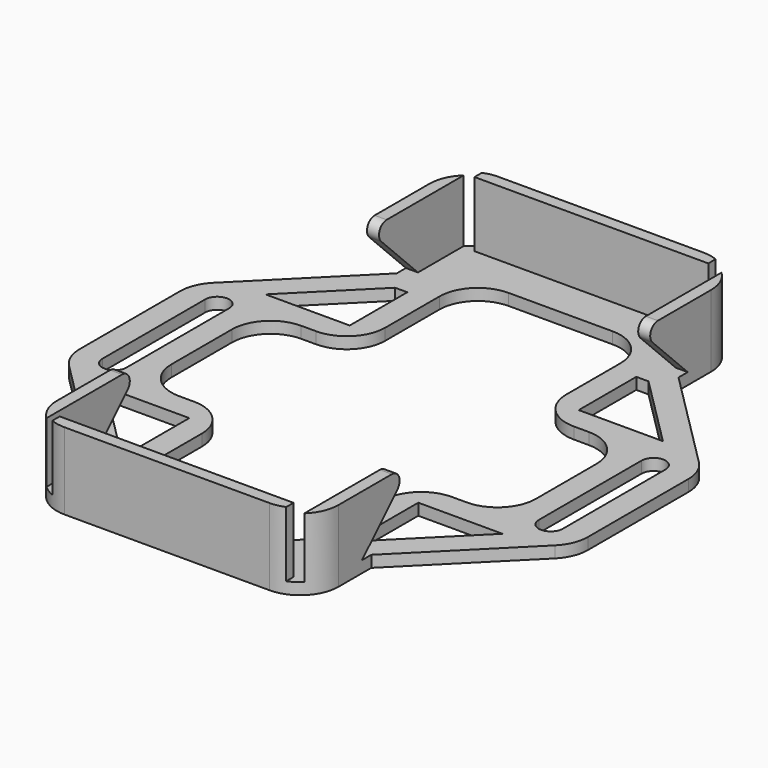
from build123d import *

# Parameters (mm, degrees)
F1_DEPTH        = 35.8775
F3_DEPTH        = 25.4
F4_W            = 1.5875
F4_H            = 8.9535
F5_DEPTH        = 9.525
F6_W            = 30.924
F6_H            = 1.5875
F5_FACE_W       = 1.5875
F5_FACE_H       = 8.9535
F7_DEPTH        = 8.636
F8_W            = 4.9497522414
F8_H            = 7.6485192403
F9_DEPTH        = 71.756
F10_W           = 23.939
F10_H           = 58.42
F11_DEPTH       = 1.525
F13_DEPTH       = 25.4
F14_W           = 12.1285
F14_H           = 20.175
F15_DEPTH       = 25.4
F16_F1_R        = 5.08
F16_F2_R        = 5.08
F16_S1_T1_DEPTH = 26.1520932665
F18_DEPTH       = 25.4
F20_DEPTH       = 1.5875
F22_DEPTH       = 1.5875
F23_R           = 1.27
F24_W           = 14.2291039228
F24_H           = 17.7929829806
F25_DEPTH       = 2.54


# Not quite as in the source:
# - a fillet or chamfer that OpenCascade refuses, or shapes differently, is made with other operations: its cross-section is extruded or revolved along the edge and cut away or added


with BuildPart() as f1:
    # F0 (on Front) → F1 (new body, symmetric)
    with BuildSketch(Plane.XZ):
        Polygon((17.875, 0.762), (-17.875, 0.762), (-18.637, 0.762), (-18.637, 0), (-18.637, -0.762), (18.637, -0.762), (18.637, 0), (18.637, 0.762), align=None)
    extrude(amount=F1_DEPTH, both=True)

    # F2 (on Front) → F3 (join, symmetric)
    with BuildSketch(Plane.XZ):
        Polygon((33.623, 0.762), (20.923, 0.762), (18.637, 0.762), (18.637, -0.762), (33.623, -0.762), align=None)
        Polygon((-18.637, 0.762), (-20.923, 0.762), (-33.623, 0.762), (-33.623, -0.762), (-18.637, -0.762), (-18.637, 0), align=None)
    extrude(amount=F3_DEPTH, both=True)

    # F4 (on face) → F5 (join)
    with BuildSketch(Plane(origin=(0, 0, -0.762), x_dir=(1, 0, 0), z_dir=(0, 0, -1))):
        with Locations((-17.84325, 31.40075)):
            Rectangle(F4_W, F4_H)
        with Locations((17.84325, 31.40075)):
            Rectangle(F4_W, F4_H)
        with Locations((-17.84325, -31.40075)):
            Rectangle(F4_W, F4_H)
        with Locations((17.84325, -31.40075)):
            Rectangle(F4_W, F4_H)
    extrude(amount=-F5_DEPTH)

    # F6 (on face) + F5_face (on face) → F7 (join)
    with BuildSketch(Plane.XY.offset(0.762)):
        with Locations((0, 35.08375)):
            Rectangle(F6_W, F6_H)
        with Locations((0, -35.08375)):
            Rectangle(F6_W, F6_H)
    with BuildSketch(Plane(origin=(-17.84325, 31.40075, 8.763), x_dir=(1, 0, 0), z_dir=(0, 0, 1))):
        Rectangle(F5_FACE_W, F5_FACE_H)
    extrude(amount=F7_DEPTH)

    # F8 (on face) → F9 (cut, through all)
    with BuildSketch(Plane(origin=(0, 35.8775, 0), x_dir=(-1, 0, 0), z_dir=(0, 1, 0))):
        with Locations((18.5586120933, 12.8226471134)):
            Rectangle(F8_W, F8_H)
    extrude(amount=-F9_DEPTH, mode=Mode.SUBTRACT)

    # F10 (on face) → F11 (cut, through all)
    with BuildSketch(Plane.XY.offset(0.762)):
        with BuildLine():
            ThreePointArc((-30.448, -8.5), (-28.8605, -10.0875), (-27.273, -8.5))
            Line((-27.273, -8.5), (-27.273, 8.5))
            ThreePointArc((-27.273, 8.5), (-28.8605, 10.0875), (-30.448, 8.5))
            Line((-30.448, 8.5), (-30.448, -8.5))
        make_face()
        with BuildLine():
            Line((27.273, 8.5), (27.273, -8.5))
            ThreePointArc((27.273, -8.5), (28.8605, -10.0875), (30.448, -8.5))
            Line((30.448, -8.5), (30.448, 8.5))
            ThreePointArc((30.448, 8.5), (28.8605, 10.0875), (27.273, 8.5))
        make_face()
        Rectangle(F10_W, F10_H)
    extrude(amount=-F11_DEPTH, mode=Mode.SUBTRACT)

    # F12 (on face) → F13 (cut)
    with BuildSketch(Plane.XY.offset(0.762)):
        Polygon((33.623, 25.4), (18.637, 25.4), (33.623, 10.414), align=None)
        Polygon((33.623, -10.414), (18.637, -25.4), (33.623, -25.4), align=None)
        Polygon((-18.637, 25.4), (-33.623, 25.4), (-33.623, 10.414), align=None)
        Polygon((-33.623, -10.414), (-33.623, -25.4), (-18.637, -25.4), align=None)
    extrude(amount=-F13_DEPTH, mode=Mode.SUBTRACT)

    # F14 (on face) → F15 (cut)
    with BuildSketch(Plane.XY.offset(0.762)):
        with Locations((-18.03375, 0)):
            Rectangle(F14_W, F14_H)
        with Locations((18.03375, 0)):
            Rectangle(F14_W, F14_H)
        Polygon((-15.1445, 16.4375), (-23.1093719395, 16.4375), (-26.2843719395, 13.2625), (-15.1445, 13.2625), align=None)
        Polygon((-19.9343719395, 19.6125), (-16.7593719395, 19.6125), (-15.1445, 19.6125), (-15.1445, 22.7875), (-16.7593719395, 22.7875), align=None)
        Polygon((16.7593719395, 19.6125), (19.9343719395, 19.6125), (16.7593719395, 22.7875), (15.1445, 22.7875), (15.1445, 19.6125), align=None)
        Polygon((23.1093719395, 16.4375), (15.1445, 16.4375), (15.1445, 13.2625), (26.2843719395, 13.2625), align=None)
        Polygon((26.2843719395, -13.2625), (15.1445, -13.2625), (15.1445, -16.4375), (23.1093719395, -16.4375), align=None)
        Polygon((16.7593719395, -22.7875), (19.9343719395, -19.6125), (16.7593719395, -19.6125), (15.1445, -19.6125), (15.1445, -22.7875), align=None)
        Polygon((-15.1445, -13.2625), (-26.2843719395, -13.2625), (-23.1093719395, -16.4375), (-15.1445, -16.4375), align=None)
        Polygon((-15.1445, -19.6125), (-16.7593719395, -19.6125), (-19.9343719395, -19.6125), (-16.7593719395, -22.7875), (-15.1445, -22.7875), align=None)
    extrude(amount=-F15_DEPTH, mode=Mode.SUBTRACT)

    # F16: fillet of radius 5.08 on 20 edges, made by hand

    # F16_f1
    f16_f1_edges = [f1.edges().sort_by_distance(p)[0] for p in [
        (-24.098, 10.0875, 0),
        (-24.098, -10.0875, 0),
        (-11.9695, 29.21, 0),
        (11.9695, 29.21, 0),
        (24.098, 10.0875, 0),
        (24.098, -10.0875, 0),
        (11.9695, -29.21, 0),
        (-11.9695, -29.21, 0),
    ]]
    fillet(f16_f1_edges, radius=F16_F1_R)

    # F16_f2
    f16_f2_edges = [f1.edges().sort_by_distance(p)[0] for p in [
        (-33.623, -10.414, 0),
        (-33.623, 10.414, 0),
        (-11.9695, -10.0875, 0),
        (-11.9695, 10.0875, 0),
        (11.9695, 10.0875, 0),
        (11.9695, -10.0875, 0),
        (33.623, -10.414, 0),
        (33.623, 10.414, 0),
        (18.637, 35.8775, 4.0005),
        (-18.637, 35.8775, 4.1181937466),
        (18.637, -35.8775, 4.0005),
        (-18.637, -35.8775, 4.0005),
    ]]
    fillet(f16_f2_edges, radius=F16_F2_R)

    # F16#s1: fillet of radius 5.08 on 1 edges, made by hand

    # F16_s1_s2 → F16_s1_t1 (cut)
    with BuildSketch(Plane.XY.offset(3.9469067335)):
        with BuildLine():
            ThreePointArc((-13.557, 35.8775), (-17.1491024484, 34.3896024484), (-18.637, 30.7975))
            Line((-18.637, 30.7975), (-18.637, 35.8775))
            Line((-18.637, 35.8775), (-13.557, 35.8775))
        make_face()
    extrude(amount=F16_S1_T1_DEPTH, mode=Mode.SUBTRACT)

    # F17 (on face) → F18 (cut)
    with BuildSketch(Plane.XY.offset(0.762)):
        Polygon((-15.1445, 19.6125), (-19.9343719395, 19.6125), (-23.1093719395, 16.4375), (-15.1445, 16.4375), align=None)
        Polygon((19.9343719395, 19.6125), (15.1445, 19.6125), (15.1445, 16.4375), (23.1093719395, 16.4375), align=None)
        Polygon((23.1093719395, -16.4375), (15.1445, -16.4375), (15.1445, -19.6125), (19.9343719395, -19.6125), align=None)
        Polygon((-15.1445, -16.4375), (-23.1093719395, -16.4375), (-19.9343719395, -19.6125), (-15.1445, -19.6125), align=None)
    extrude(amount=-F18_DEPTH, mode=Mode.SUBTRACT)

    # F19 (on face) → F20 (join)
    with BuildSketch(Plane.YZ.offset(18.637)):
        Polygon((18.923, 8.763), (26.924, 0.762), (26.924, 8.763), align=None)
        Polygon((-26.924, 8.763), (-26.924, 0.762), (-18.923, 8.763), align=None)
    extrude(amount=-F20_DEPTH)

    # F21 (on face) → F22 (join)
    with BuildSketch(Plane(origin=(-18.637, 0, 0), x_dir=(0, -1, 0), z_dir=(-1, 0, 0))):
        Polygon((18.923, 8.763), (26.924, 0.762), (26.924, 8.763), align=None)
        Polygon((-26.924, 8.9983874932), (-26.924, 0.762), (-18.6876125068, 8.9983874932), align=None)
    extrude(amount=-F22_DEPTH)

    # F23
    f23_edges = [f1.edges().sort_by_distance(p)[0] for p in [
        (-17.84325, 18.687613, 8.998387),
        (-17.84325, -18.923, 8.763),
        (17.84325, -18.923, 8.763),
        (17.84325, 18.923, 8.763),
    ]]
    fillet(f23_edges, radius=F23_R)

    # F24 (on face) → F25 (cut)
    with BuildSketch(Plane.XY.offset(17.399)):
        with Locations((-13.9599367976, 29.4290939346)):
            Rectangle(F24_W, F24_H)
    extrude(amount=-F25_DEPTH, mode=Mode.SUBTRACT)


solid = f1.part
